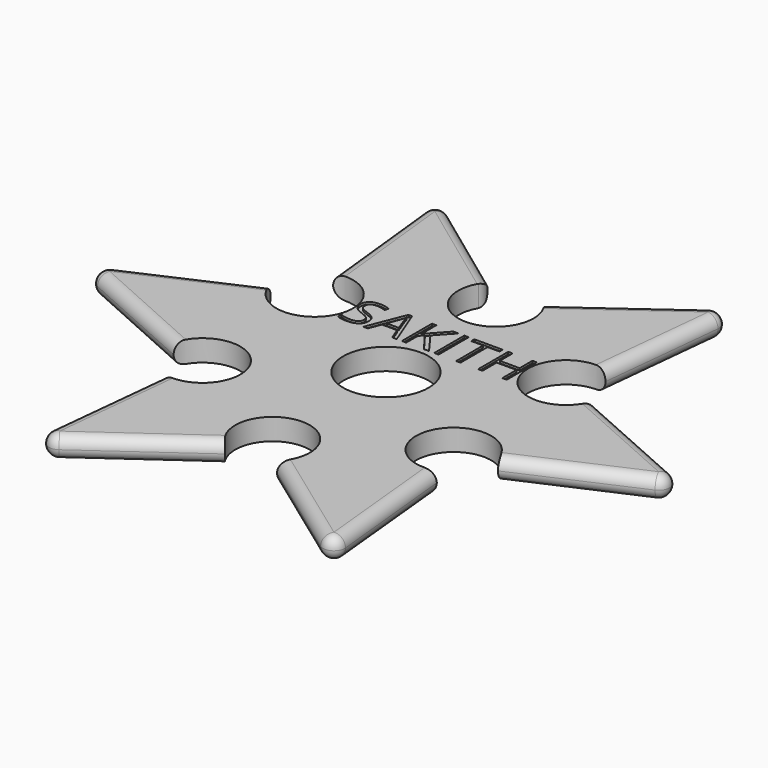
from build123d import *

# Parameters (mm, degrees)
F0_R         = 5.0393871199
F1_DEPTH     = 2.54
F2_TEXT_SIZE = 6.2250579888
F3_DEPTH     = 0.254
F4_R         = 1.26999


# Not quite as in the source:
# - a fillet or chamfer is up to 0.001 mm smaller than in the source, because OpenCascade refuses the exact size
# - Text() gives the source's letters only with a copy of the font that has no kerning and outlines rounded to 1/6400 em; it was checked with that copy


with BuildPart() as f1:
    # F0 (on Top) → F1 (new body)
    with BuildSketch(Plane.XY):
        with BuildLine():
            Line((18.8024565578, 61.6474449635), (20.7559820265, 43.4293486178))
            ThreePointArc((20.7559820265, 43.4293486178), (25.9431089283, 36.794298763), (17.6274608821, 38.128528744))
            Line((17.6274608821, 38.128528744), (1.3515243772, 30.8491047472))
            Line((1.3515243772, 30.8491047472), (17.9284568876, 23.4276503325))
            ThreePointArc((17.9284568876, 23.4276503325), (26.1219882102, 24.5149583107), (21.0390482098, 17.997296527))
            Line((21.0390482098, 17.997296527), (19.2277058959, 0.4166367871))
            Line((19.2277058959, 0.4166367871), (33.9986681938, 10.9416656196))
            ThreePointArc((33.9986681938, 10.9416656196), (37.0598398149, 18.5041104915), (40.121011436, 10.9416656196))
            Line((40.121011436, 10.9416656196), (54.6485595405, 0.4166367871))
            Line((54.6485595405, 0.4166367871), (52.8354048729, 18.615482375))
            ThreePointArc((52.8354048729, 18.615482375), (47.5401445847, 24.9468801366), (55.7403787971, 24.0074452013))
            Line((55.7403787971, 24.0074452013), (72.0529779792, 31.2268864363))
            Line((72.0529779792, 31.2268864363), (55.4822795093, 38.595225662))
            ThreePointArc((55.4822795093, 38.595225662), (47.2616721513, 37.5739519936), (52.3492731154, 44.1113598645))
            Line((52.3492731154, 44.1113598645), (54.1418157518, 61.6474449635))
            Line((54.1418157518, 61.6474449635), (39.5202822983, 51.0497204959))
            ThreePointArc((39.5202822983, 51.0497204959), (36.3738108426, 43.4749513334), (33.2273393869, 51.0497204959))
            Line((33.2273393869, 51.0497204959), (18.8024565578, 61.6474449635))
        make_face()
        with Locations((36.8770882487, 31.0666156864)):
            Circle(F0_R, mode=Mode.SUBTRACT)
    extrude(amount=F1_DEPTH)

    # F2 (on face) → F3 (cut)
    with BuildSketch(Plane.XY.offset(2.54)):
        with Locations((26.190951002, 36.8087053297)):
            Text('SAKITH', F2_TEXT_SIZE, font='Open Sans', text_align=(TextAlign.LEFT, TextAlign.BOTTOM))
    extrude(amount=-F3_DEPTH, mode=Mode.SUBTRACT)

    # F4 (radius 1.27 in the source; OpenCascade refuses exactly that, so slightly less here)
    f4_edges = [f1.edges().sort_by_distance(p)[0] for p in [
        (26.014898, 56.348583, 2.54),
        (26.014898, 56.348583, 0),
        (19.779219, 52.538397, 2.54),
        (19.779219, 52.538397, 0),
        (33.227339, 51.04972, 1.27),
        (18.802457, 61.647445, 1.27),
        (9.639991, 27.138378, 0),
        (9.639991, 27.138378, 2.54),
        (1.351524, 30.849105, 1.27),
        (9.489493, 34.488817, 2.54),
        (9.489493, 34.488817, 0),
        (19.227706, 0.416637, 1.27),
        (20.133377, 9.206967, 0),
        (20.133377, 9.206967, 2.54),
        (26.613187, 5.679151, 0),
        (26.613187, 5.679151, 2.54),
        (47.384785, 5.679151, 0),
        (54.64856, 0.416637, 1.27),
        (47.384785, 5.679151, 2.54),
        (53.741982, 9.51606, 0),
        (53.741982, 9.51606, 2.54),
        (63.896678, 27.617166, 2.54),
        (63.896678, 27.617166, 0),
        (72.052978, 31.226886, 1.27),
        (63.767629, 34.911056, 2.54),
        (63.767629, 34.911056, 0),
        (46.831049, 56.348583, 0),
        (53.245544, 52.879402, 2.54),
        (54.141816, 61.647445, 1.27),
        (53.245544, 52.879402, 0),
        (46.831049, 56.348583, 2.54),
    ]]
    fillet(f4_edges, radius=F4_R)


solid = f1.part
